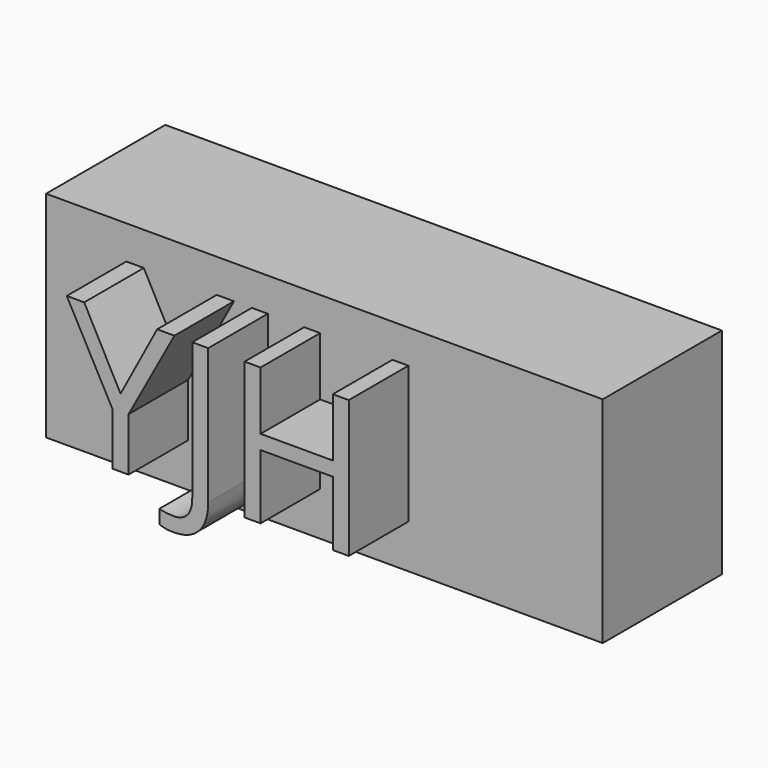
from build123d import *

# Parameters (mm, degrees)
F0_W         = 94.9073582888
F0_H         = 36.5944355726
F1_DEPTH     = 25.4
F2_TEXT_SIZE = 32.7741953596
F3_DEPTH     = 12.7


# Not quite as in the source:
# - Text() gives the source's letters only with a copy of the font that has no kerning and outlines rounded to 1/6400 em; it was checked with that copy


with BuildPart() as f1:
    # F0 (on Front) → F1 (new body)
    with BuildSketch(Plane.XZ):
        with Locations((47.4536791444, 18.2972177863)):
            Rectangle(F0_W, F0_H)
    extrude(amount=F1_DEPTH)

    # F2 (on face) → F3 (join)
    with BuildSketch(Plane.XZ.offset(25.4)):
        with Locations((13.6860171333, 7.4663707055)):
            Text('YJH', F2_TEXT_SIZE, font='Open Sans', text_align=(TextAlign.LEFT, TextAlign.BOTTOM))
    extrude(amount=F3_DEPTH)


solid = f1.part
